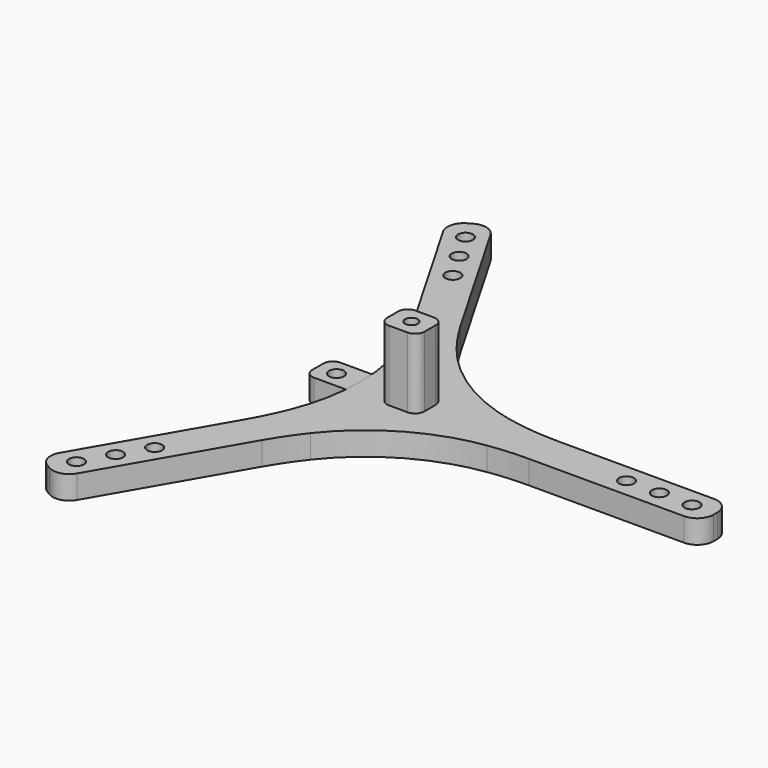
from build123d import *

# Parameters (mm, degrees)
F0_W      = 40
F0_H      = 7
F0_R      = 1.6
F0_R_2    = 1.35
F1_DEPTH  = 5
F2_W      = 8
F2_H      = 7
F2_R      = 1.35
F3_DEPTH  = 20
F4_R      = 2
F5_R      = 1.6
F6_DEPTH  = 5
F7_R      = 60
F8_R      = 3.5
F10_COUNT = 3
F11_R     = 40


with BuildPart() as f1:
    # F0 (on Top) → F1 (new body)
    with BuildSketch(Plane.XY):
        Rectangle(F0_W, F0_H)
        with Locations((-16, 0)):
            Circle(F0_R, mode=Mode.SUBTRACT)
        with Locations((-9, 0)):
            Circle(F0_R, mode=Mode.SUBTRACT)
        Circle(F0_R_2, mode=Mode.SUBTRACT)
        with Locations((9, 0)):
            Circle(F0_R, mode=Mode.SUBTRACT)
        with Locations((16, 0)):
            Circle(F0_R, mode=Mode.SUBTRACT)
    extrude(amount=F1_DEPTH)

    # F2 (on Top) → F3 (join)
    with BuildSketch(Plane.XY):
        Rectangle(F2_W, F2_H)
        Circle(F2_R, mode=Mode.SUBTRACT)
    extrude(amount=F3_DEPTH)

    # F4
    f4_edges = [f1.edges().sort_by_distance(p)[0] for p in [
        (-20, -3.5, 2.5),
        (-20, 3.5, 2.5),
        (20, -3.5, 2.5),
        (-4, -3.5, 12.5),
        (4, -3.5, 12.5),
        (-4, 3.5, 12.5),
        (20, 3.5, 2.5),
        (4, 3.5, 12.5),
    ]]
    fillet(f4_edges, radius=F4_R)


with BuildPart() as f6:
    # F5 (on Top) → F6 (new body)
    with BuildSketch(Plane.XY):
        with BuildLine():
            Line((0, -4), (0, 4))
            Line((0, 4), (9.1651513899, 4))
            ThreePointArc((9.1651513899, 4), (-10, 0), (9.1651513899, -4))
            Line((9.1651513899, -4), (0, -4))
        make_face()
        with BuildLine():
            Line((9.1651513899, 4), (0, 4))
            Line((0, 4), (0, -4))
            Line((0, -4), (9.1651513899, -4))
            ThreePointArc((9.1651513899, -4), (9.7890631293, -2.0430964369), (10, 0))
            ThreePointArc((10, 0), (9.7890631293, 2.0430964369), (9.1651513899, 4))
        make_face()
        with BuildLine():
            Line((65, 4), (9.1651513899, 4))
            ThreePointArc((9.1651513899, 4), (9.7890631293, 2.0430964369), (10, 0))
            ThreePointArc((10, 0), (9.7890631293, -2.0430964369), (9.1651513899, -4))
            Line((9.1651513899, -4), (65, -4))
            Line((65, -4), (65, 4))
        make_face()
        with Locations((46, 0)):
            Circle(F5_R, mode=Mode.SUBTRACT)
        with Locations((53, 0)):
            Circle(F5_R, mode=Mode.SUBTRACT)
        with Locations((60, 0)):
            Circle(F5_R, mode=Mode.SUBTRACT)
    extrude(amount=F6_DEPTH)

    # F7
    f7_edges = [f6.edges().sort_by_distance(p)[0] for p in [
        (9.165151, -4, 2.5),
        (9.165151, 4, 2.5),
    ]]
    fillet(f7_edges, radius=F7_R)

    # F8
    f8_edges = [f6.edges().sort_by_distance(p)[0] for p in [
        (65, -4, 2.5),
        (65, 4, 2.5),
    ]]
    fillet(f8_edges, radius=F8_R)

    # F10: F6 ×3 about axis
    f10_axis = Axis((0, 0, 9.6070729196), (0, 0, 1))


with BuildPart() as f6_1:
    add(f6.part)
    for i in range(1, F10_COUNT):
        add(f6.part.rotate(f10_axis, i * 360 / F10_COUNT))

    # F11
    f11_edges = [f6_1.edges().sort_by_distance(p)[0] for p in [
        (5.033316, -8.717959, 2.5),
        (-10.066632, 0, 2.5),
        (5.033316, 8.717959, 2.5),
    ]]
    fillet(f11_edges, radius=F11_R)


solid = Compound([f1.part, f6_1.part])
